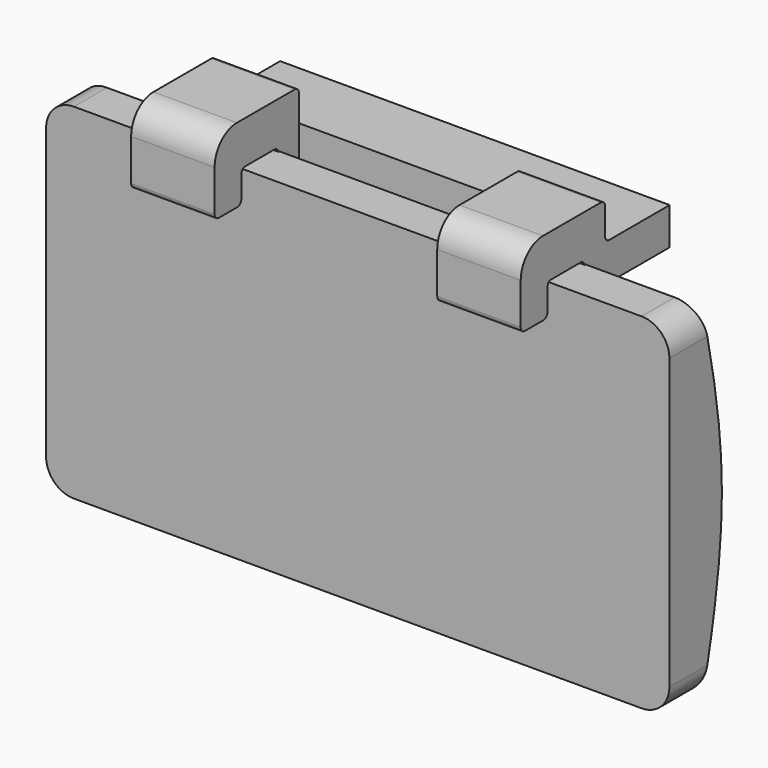
from build123d import *

# Parameters (mm, degrees)
F1_DEPTH      = 14.986
F3_DEPTH      = 142.241
F5_DEPTH      = 44.45
F5_DEPTH_BACK = 44.45
F6_DEPTH      = 25.4
F6_DEPTH_BACK = 25.4


# Not quite as in the source:
# - a feature names something its author has since deleted; it is built from what else it names


with BuildPart() as f1:
    # F0 (on Front) → F1 (new body)
    with BuildSketch(Plane.XZ):
        with BuildLine():
            Line((-64.77, -39.37), (64.77, -39.37))
            ThreePointArc((64.77, -39.37), (69.2601280605, -37.5101280605), (71.12, -33.02))
            Line((71.12, -33.02), (71.12, 33.02))
            ThreePointArc((71.12, 33.02), (69.2601280605, 37.5101280605), (64.77, 39.37))
            Line((64.77, 39.37), (-64.77, 39.37))
            ThreePointArc((-64.77, 39.37), (-69.2601280605, 37.5101280605), (-71.12, 33.02))
            Line((-71.12, 33.02), (-71.12, -33.02))
            ThreePointArc((-71.12, -33.02), (-69.2601280605, -37.5101280605), (-64.77, -39.37))
        make_face()
    extrude(amount=F1_DEPTH)

    # F2 (on face) → F3 (cut, through all)
    with BuildSketch(Plane.YZ.offset(71.12)):
        with BuildLine():
            Line((0, 39.37), (-5.588, 39.37))
            add(Edge.make_bspline(
                [(-5.588, 39.37), (-5.0939327167, 37.2564899548), (-4.6132131193, 35.139642988), (-4.1544956107, 33.02)],
                knots=[0, 0, 0, 0, 0.0810477827, 0.0810477827, 0.0810477827, 0.0810477827], degree=3))
            Line((-4.1544956107, 33.02), (0, 33.02))
            Line((0, 33.02), (0, 39.37))
        make_face()
        with BuildLine():
            Line((0, 33.02), (-4.1544956107, 33.02))
            add(Edge.make_bspline(
                [(-4.1544956107, 33.02), (-1.7832929575, 22.0631409692), (0, 11.0315704846), (0, 0)],
                knots=[0.0810477827, 0.0810477827, 0.0810477827, 0.0810477827, 0.5, 0.5, 0.5, 0.5], degree=3))
            Line((0, 0), (0, 33.02))
        make_face()
        with BuildLine():
            Line((0, -33.02), (0, 0))
            add(Edge.make_bspline(
                [(0, 0), (0, -11.0315704846), (-1.7832929575, -22.0631409692), (-4.1544956107, -33.02)],
                knots=[0.5, 0.5, 0.5, 0.5, 0.9189522173, 0.9189522173, 0.9189522173, 0.9189522173], degree=3))
            Line((-4.1544956107, -33.02), (0, -33.02))
        make_face()
        with BuildLine():
            Line((0, -33.02), (-4.1544956107, -33.02))
            add(Edge.make_bspline(
                [(-4.1544956107, -33.02), (-4.6132131193, -35.139642988), (-5.0939327167, -37.2564899548), (-5.588, -39.37)],
                knots=[0.9189522173, 0.9189522173, 0.9189522173, 0.9189522173, 1, 1, 1, 1], degree=3))
            Line((-5.588, -39.37), (0, -39.37))
            Line((0, -39.37), (0, -39.1186140473))
            Line((0, -39.1186140473), (0, -33.02))
        make_face()
    extrude(amount=-F3_DEPTH, mode=Mode.SUBTRACT)


with BuildPart() as f5:
    # F4 (on Right) → F5 (new body, two sides)
    with BuildSketch(Plane.YZ) as f5_sk:
        with BuildLine():
            Line((-1.2158148456, 50.0348769128), (-17.7066842258, 50.0348769128))
            ThreePointArc((-17.7066842258, 50.0348769128), (-22.1968122863, 48.1750049734), (-24.0566842258, 43.6848769128))
            Line((-24.0566842258, 43.6848769128), (-24.0566842258, 34.2530116905))
            ThreePointArc((-24.0566842258, 34.2530116905), (-23.7005803022, 33.3933007684), (-22.8408693802, 33.0371968448))
            Line((-22.8408693802, 33.0371968448), (-17.6238791954, 33.0371968448))
            ThreePointArc((-17.6238791954, 33.0371968448), (-16.7641682733, 33.3933007684), (-16.4080643497, 34.2530116905))
            Line((-16.4080643497, 34.2530116905), (-16.4080643497, 39.3098837759))
            ThreePointArc((-16.4080643497, 39.3098837759), (-16.1104848394, 40.0283042656), (-15.3920643497, 40.3258837759))
            Line((-15.3920643497, 40.3258837759), (-7.023171001, 40.3258837759))
            ThreePointArc((-7.023171001, 40.3258837759), (-6.2922111741, 40.0816158774), (-5.8549638669, 39.4469633211))
            Line((-5.8549638669, 39.4469633211), (-4.2599462141, 33.9161172996))
            ThreePointArc((-4.2599462141, 33.9161172996), (-3.8226989069, 33.2814647434), (-3.09173908, 33.0371968448))
            Line((-3.09173908, 33.0371968448), (0, 33.0371968448))
            Line((0, 33.0371968448), (0, 41.5360368788))
            Line((0, 41.5360368788), (0, 42.7518517245))
            Line((0, 42.7518517245), (0, 44.9006222188))
            Line((0, 44.9006222188), (0, 48.8190620672))
            ThreePointArc((0, 48.8190620672), (-0.3561039236, 49.6787729892), (-1.2158148456, 50.0348769128))
        make_face()
        with BuildLine():
            ThreePointArc((1.2158148456, 41.5360368788), (0.3561039236, 41.8921408024), (0, 42.7518517245))
            Line((0, 42.7518517245), (0, 41.5360368788))
            Line((0, 41.5360368788), (1.2158148456, 41.5360368788))
        make_face()
        Polygon((18.4375178069, 41.5360368788), (1.2158148456, 41.5360368788), (0, 41.5360368788), (0, 33.0371968448), (18.4375178069, 33.0371968448), align=None)
    extrude(amount=F5_DEPTH)
    extrude(f5_sk.sketch, amount=-F5_DEPTH_BACK)

    # F4 (on Right) → F6 (cut, two sides)
    with BuildSketch(Plane.YZ) as f6_sk:
        with BuildLine():
            Line((-1.2158148456, 50.0348769128), (-17.7066842258, 50.0348769128))
            ThreePointArc((-17.7066842258, 50.0348769128), (-22.1968122863, 48.1750049734), (-24.0566842258, 43.6848769128))
            Line((-24.0566842258, 43.6848769128), (-24.0566842258, 34.2530116905))
            ThreePointArc((-24.0566842258, 34.2530116905), (-23.7005803022, 33.3933007684), (-22.8408693802, 33.0371968448))
            Line((-22.8408693802, 33.0371968448), (-17.6238791954, 33.0371968448))
            ThreePointArc((-17.6238791954, 33.0371968448), (-16.7641682733, 33.3933007684), (-16.4080643497, 34.2530116905))
            Line((-16.4080643497, 34.2530116905), (-16.4080643497, 39.3098837759))
            ThreePointArc((-16.4080643497, 39.3098837759), (-16.1104848394, 40.0283042656), (-15.3920643497, 40.3258837759))
            Line((-15.3920643497, 40.3258837759), (-7.023171001, 40.3258837759))
            ThreePointArc((-7.023171001, 40.3258837759), (-6.2922111741, 40.0816158774), (-5.8549638669, 39.4469633211))
            Line((-5.8549638669, 39.4469633211), (-4.2599462141, 33.9161172996))
            ThreePointArc((-4.2599462141, 33.9161172996), (-3.8226989069, 33.2814647434), (-3.09173908, 33.0371968448))
            Line((-3.09173908, 33.0371968448), (0, 33.0371968448))
            Line((0, 33.0371968448), (0, 41.5360368788))
            Line((0, 41.5360368788), (0, 42.7518517245))
            Line((0, 42.7518517245), (0, 44.9006222188))
            Line((0, 44.9006222188), (0, 48.8190620672))
            ThreePointArc((0, 48.8190620672), (-0.3561039236, 49.6787729892), (-1.2158148456, 50.0348769128))
        make_face()
    extrude(amount=-F6_DEPTH, mode=Mode.SUBTRACT)
    extrude(f6_sk.sketch, amount=F6_DEPTH_BACK, mode=Mode.SUBTRACT)


solid = Compound([f1.part, f5.part])
